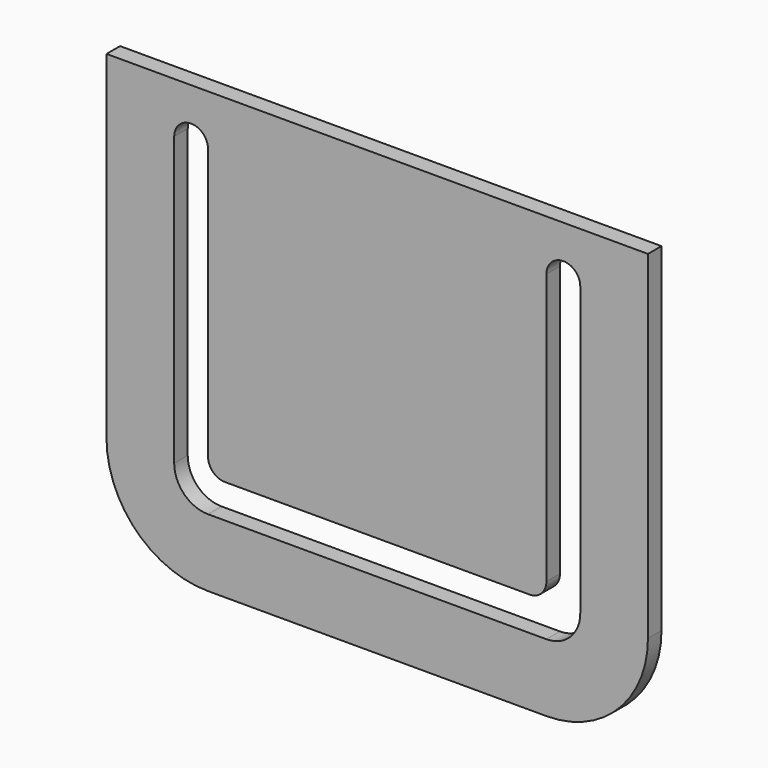
from build123d import *

# Parameters (mm, degrees)
F0_W      = 25.4
F0_H      = 19.05
F1_DEPTH  = 0.79375
F2_R      = 4.7625
F3_W      = 19.05
F3_H      = 15.875
F4_DEPTH  = 4.9276
F6_DEPTH  = 0.79375
F7_R      = 1.5875
F9_W      = 15.875
F9_H      = 14.2875
F10_DEPTH = 0.79375
F11_R     = 0.79374
F12_R     = 0.79375
F14_DEPTH = 25.4
F15_W     = 25.4
F15_H     = 4.7625
F16_DEPTH = 25.4


# Not quite as in the source:
# - two fillets or chamfers of one size are made in one step
# - a fillet or chamfer is up to 0.001 mm smaller than in the source, because OpenCascade refuses the exact size


with BuildPart() as f1:
    # F0 (on Front) → F1 (new body)
    with BuildSketch(Plane.XZ):
        Rectangle(F0_W, F0_H)
    extrude(amount=F1_DEPTH)

    # F2
    f2_edges = [f1.edges().sort_by_distance(p)[0] for p in [
        (12.7, -0.396875, -9.525),
        (-12.7, -0.396875, -9.525),
    ]]
    fillet(f2_edges, radius=F2_R)

    # F3 (on face) → F4 (cut)
    with BuildSketch(Plane.XZ.offset(0.79375)):
        with Locations((0, 1.5875)):
            Rectangle(F3_W, F3_H)
    extrude(amount=-F4_DEPTH, mode=Mode.SUBTRACT)

    # F5 (on face) → F6 (join)
    with BuildSketch(Plane.XZ.offset(0.79375)):
        Polygon((-15.875, 15.875), (-15.875, 9.525), (-12.7, 9.525), (-9.525, 9.525), (9.525, 9.525), (12.7, 9.525), (15.875, 9.525), (15.875, 15.875), align=None)
    extrude(amount=-F6_DEPTH)

    # F7
    f7_edges = [f1.edges().sort_by_distance(p)[0] for p in [
        (-15.875, -0.396875, 15.875),
        (15.875, -0.396875, 15.875),
        (15.875, -0.396875, 9.525),
        (-15.875, -0.396875, 9.525),
        (-9.525, -0.396875, -6.35),
        (9.525, -0.396875, -6.35),
    ]]
    fillet(f7_edges, radius=F7_R)

    # F9 (on face) → F10 (join)
    with BuildSketch(Plane.XZ.offset(0.79375)):
        with BuildLine():
            ThreePointArc((-14.2875, 15.875), (-15.4100320151, 15.4100320151), (-15.875, 14.2875))
            Line((-15.875, 14.2875), (-15.875, 11.1125))
            ThreePointArc((-15.875, 11.1125), (-15.4100320151, 9.9899679849), (-14.2875, 9.525))
            Line((-14.2875, 9.525), (-12.7, 9.525))
            Line((-12.7, 9.525), (-12.7, -4.7625))
            ThreePointArc((-12.7, -4.7625), (-11.3050960454, -8.1300960454), (-7.9375, -9.525))
            Line((-7.9375, -9.525), (7.9375, -9.525))
            ThreePointArc((7.9375, -9.525), (11.3050960454, -8.1300960454), (12.7, -4.7625))
            Line((12.7, -4.7625), (12.7, 9.525))
            Line((12.7, 9.525), (14.2875, 9.525))
            ThreePointArc((14.2875, 9.525), (15.4100320151, 9.9899679849), (15.875, 11.1125))
            Line((15.875, 11.1125), (15.875, 14.2875))
            ThreePointArc((15.875, 14.2875), (15.4100320151, 15.4100320151), (14.2875, 15.875))
            Line((14.2875, 15.875), (-14.2875, 15.875))
        make_face()
        with BuildLine():
            Line((-9.525, 9.525), (-7.9375, 9.525))
            Line((-7.9375, 9.525), (7.9375, 9.525))
            Line((7.9375, 9.525), (9.525, 9.525))
            Line((9.525, 9.525), (9.525, -4.7625))
            ThreePointArc((9.525, -4.7625), (9.0600320151, -5.8850320151), (7.9375, -6.35))
            Line((7.9375, -6.35), (-7.9375, -6.35))
            ThreePointArc((-7.9375, -6.35), (-9.0600320151, -5.8850320151), (-9.525, -4.7625))
            Line((-9.525, -4.7625), (-9.525, 9.525))
        make_face(mode=Mode.SUBTRACT)
        with Locations((0, 2.38125)):
            Rectangle(F9_W, F9_H)
    extrude(amount=-F10_DEPTH)

    # F11 (radius 0.79375 in the source; OpenCascade refuses exactly that, so slightly less here)
    f11_edges = [f1.edges().sort_by_distance(p)[0] for p in [
        (-7.9375, -0.396875, 9.525),
        (-9.525, -0.396875, 9.525),
        (7.9375, -0.396875, 9.525),
        (9.525, -0.396875, 9.525),
    ]]
    fillet(f11_edges, radius=F11_R)

    # F12
    f12_edges = [f1.edges().sort_by_distance(p)[0] for p in [
        (-7.9375, -0.396875, -4.7625),
        (7.9375, -0.396875, -4.7625),
    ]]
    fillet(f12_edges, radius=F12_R)

    # F13 (on face) → F14 (cut)
    with BuildSketch(Plane.XZ.offset(0.79375)):
        with BuildLine():
            Line((-17.2636155039, 7.9375), (-12.7, 7.9375))
            Line((-12.7, 7.9375), (-12.7, 9.525))
            Line((-12.7, 9.525), (-14.2875, 9.525))
            ThreePointArc((-14.2875, 9.525), (-15.4100320151, 9.9899679849), (-15.875, 11.1125))
            Line((-15.875, 11.1125), (-15.875, 14.2875))
            ThreePointArc((-15.875, 14.2875), (-15.4100320151, 15.4100320151), (-14.2875, 15.875))
            Line((-14.2875, 15.875), (-12.7, 15.875))
            Line((-12.7, 15.875), (-12.7, 16.6596230119))
            Line((-12.7, 16.6596230119), (-17.2636155039, 16.6596230119))
            Line((-17.2636155039, 16.6596230119), (-17.2636155039, 7.9375))
        make_face()
        with BuildLine():
            Line((-14.2875, 9.525), (-12.7, 9.525))
            Line((-12.7, 9.525), (-12.7, 15.875))
            Line((-12.7, 15.875), (-14.2875, 15.875))
            ThreePointArc((-14.2875, 15.875), (-15.4100320151, 15.4100320151), (-15.875, 14.2875))
            Line((-15.875, 14.2875), (-15.875, 11.1125))
            ThreePointArc((-15.875, 11.1125), (-15.4100320151, 9.9899679849), (-14.2875, 9.525))
        make_face()
        with BuildLine():
            Line((14.2875, 15.875), (12.7, 15.875))
            Line((12.7, 15.875), (12.7, 9.525))
            Line((12.7, 9.525), (14.2875, 9.525))
            ThreePointArc((14.2875, 9.525), (15.4100320151, 9.9899679849), (15.875, 11.1125))
            Line((15.875, 11.1125), (15.875, 14.2875))
            ThreePointArc((15.875, 14.2875), (15.4100320151, 15.4100320151), (14.2875, 15.875))
        make_face()
        with BuildLine():
            Line((12.7, 16.9361550361), (12.7, 15.875))
            Line((12.7, 15.875), (14.2875, 15.875))
            ThreePointArc((14.2875, 15.875), (15.4100320151, 15.4100320151), (15.875, 14.2875))
            Line((15.875, 14.2875), (15.875, 11.1125))
            ThreePointArc((15.875, 11.1125), (15.4100320151, 9.9899679849), (14.2875, 9.525))
            Line((14.2875, 9.525), (12.7, 9.525))
            Line((12.7, 9.525), (12.7, 7.9375))
            Line((12.7, 7.9375), (16.7191289365, 7.9375))
            Line((16.7191289365, 7.9375), (16.7191289365, 16.9361550361))
            Line((16.7191289365, 16.9361550361), (12.7, 16.9361550361))
        make_face()
    extrude(amount=-F14_DEPTH, mode=Mode.SUBTRACT)

    # F15 (on face) → F16 (cut)
    with BuildSketch(Plane.XZ.offset(0.79375)):
        with Locations((0, 13.49375)):
            Rectangle(F15_W, F15_H)
    extrude(amount=-F16_DEPTH, mode=Mode.SUBTRACT)


solid = f1.part
